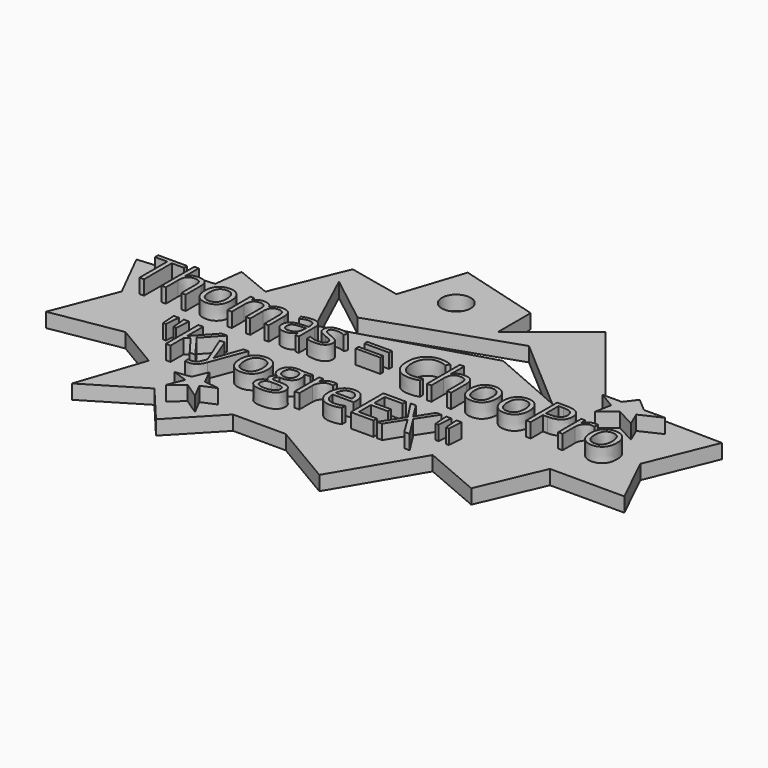
from build123d import *

# Parameters (mm, degrees)
F1_DEPTH       = 3
F2_TEXT_SIZE   = 11.251442599
F2_TEXT_SIZE_2 = 11.8668939536
F3_DEPTH       = 3
F5_DEPTH       = 3
F7_DEPTH       = 3
F8_R           = 3
F9_DEPTH       = 3
F11_DEPTH      = 3


# Not quite as in the source:
# - Text() gives the source's letters only with a copy of the font that has no kerning and outlines rounded to 1/6400 em; it was checked with that copy


with BuildPart() as f1:
    # F0 (on Top) → F1 (new body)
    with BuildSketch(Plane.XY):
        Polygon((-33.5516285011, 22.8029673027), (-34.2760205269, 16.8468564749), (-49.6074073017, 15.5595736578), (-44.4471426308, 5.2758231759), (-49.5851822197, -7.9445922747), (-35.050239414, -5.4881675169), (-25.8316509426, -10.9724104404), (-30.5374307213, -24.9937793324), (-18.9993806183, -18.0387541652), (-12.04097128, -26.3211339445), (-3.3331995963, -17.2033522278), (7.6300101834, -17.2033522278), (20.8602522535, -25.0198796065), (30.8655224741, -8.0849748105), (43.0655473261, -13.3084317695), (48.7635701895, 0), (64.2281994224, 0), (59.1064840555, 10.5395456776), (64.8522153497, 24.565892294), (40.2943715453, 24.9609742314), (25.7266242246, 43.2279115794), (12.126551941, 32.3819546029), (12.126551941, 40.809978233), (-4.7413482098, 45.5413078889), (-9.0480465442, 32.3819546029), (-20.0540525839, 34.7745632753), (-26.2085164534, 19.7875045262), align=None)
    extrude(amount=F1_DEPTH)

    # F2 (on face) → F3 (join)
    with BuildSketch(Plane.XY.offset(3)):
        with Locations((-44.2648604512, 6.3834697574)):
            Text('Thomas = ChooPro', F2_TEXT_SIZE, font='Open Sans', text_align=(TextAlign.LEFT, TextAlign.BOTTOM))
        with Locations((-29.6897493761, -9.1163676624)):
            Text('"KyogreEX"', F2_TEXT_SIZE_2, font='Open Sans', text_align=(TextAlign.LEFT, TextAlign.BOTTOM))
    extrude(amount=F3_DEPTH)

    # F4 (on face) → F5 (cut, through all)
    with BuildSketch(Plane.XY.offset(3)):
        Polygon((-8.8492082432, 22.0429431647), (-19.0778377084, 30), (-12.4013237655, 15.5262751505), (19.1336832941, 24.8920994308), (34.7998688799, 18.0744080908), (19.1336832941, 31.5888673067), align=None)
    extrude(amount=-F5_DEPTH, mode=Mode.SUBTRACT)

    # F6 (on face) → F7 (join)
    with BuildSketch(Plane.XY.offset(3)):
        Polygon((-11.9930589572, -12.5042982399), (-13.2728560746, -15.5514329672), (-16.4804282957, -15.9696675837), (-13.367257081, -17.0451272279), (-14.7414552048, -20.3910004348), (-11.9930589572, -18.1647401136), (-8.6822095443, -20.3910004348), (-10.3201223537, -17.2243695706), (-7.3924828321, -15.9696675837), (-10.4993656278, -15.5514329672), align=None)
    extrude(amount=F7_DEPTH)

    # F8 (on face) → F9 (cut, through all)
    with BuildSketch(Plane.XY.offset(3)):
        with Locations((0.5, 36)):
            Circle(F8_R)
    extrude(amount=-F9_DEPTH, mode=Mode.SUBTRACT)

    # F10 (on face) → F11 (join)
    with BuildSketch(Plane.XY.offset(3)):
        Polygon((51.3706691563, 21.1762785912), (48.5734814756, 23.5487968848), (46.7442073852, 21.1762785912), (42.7475385368, 21.1762785912), (46.154204756, 19.1535688937), (45.5154553056, 15.7469008118), (48.7092062831, 18.3019023389), (52.6481680572, 16.1727350205), (51.3706691563, 19.1535688937), (55.7373456452, 21.2045421164), align=None)
    extrude(amount=F11_DEPTH)


solid = f1.part
